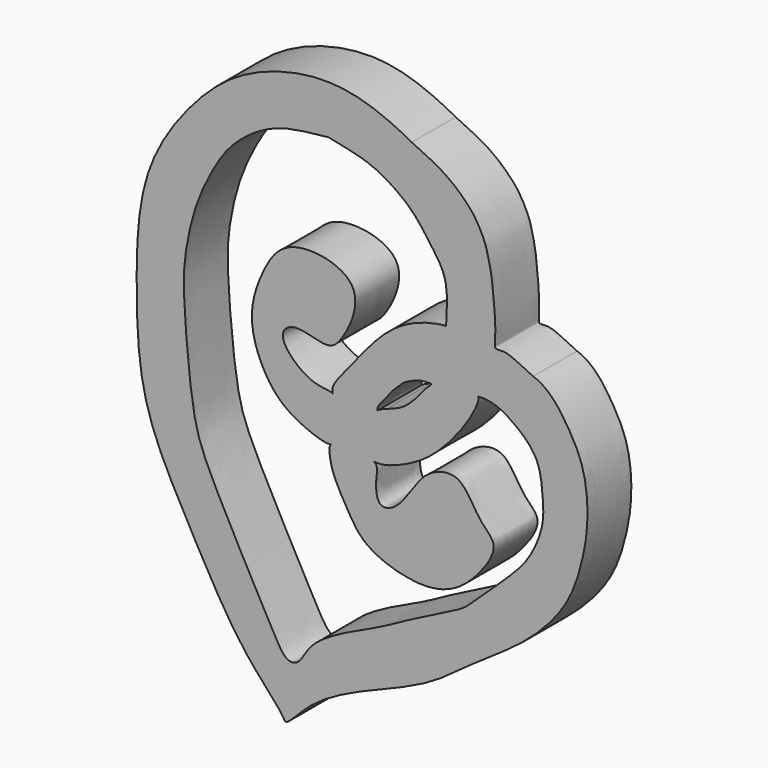
from build123d import *

# Parameters (mm, degrees)
F1_DEPTH = 5.08


with BuildPart() as f1:
    # F0 (on Front) → F1 (new body)
    with BuildSketch(Plane.XZ):
        with BuildLine():
            add(Edge.make_bspline(
                [(12.9434475675, 7.9712104052), (13.7422922583, 7.0552895324), (15.383850226, 7.4895155838), (16.7147424072, 7.0660994388)],
                knots=[0, 0, 0, 0, 0.032523755, 0.032523755, 0.032523755, 0.032523755], degree=3))
            add(Edge.make_bspline(
                [(5.4742157617, 22.5000154136), (7.1555189659, 21.5835338766), (10.6079264327, 19.2692823236), (12.792965037, 16.3012717327), (11.8126951939, 9.2676823139), (12.9434475675, 7.9712104052)],
                knots=[0.8891292206, 0.8891292206, 0.8891292206, 0.8891292206, 0.9190816899, 0.953963125, 1, 1, 1, 1], degree=3))
            add(Edge.make_bspline(
                [(16.7147424072, 7.0660994388), (18.1705162912, 6.6029528559), (20.2002028353, 3.814582201), (21.6276154231, 0.7024454413), (21.878625851, -3.3195361715), (21.2433984405, -6.8677651224), (19.8929255019, -10.9606617131), (15.8219732338, -15.1508443216), (11.9059849161, -17.5286027662), (8.1819090495, -20.4691639784), (4.3745709963, -22.4656705166), (-3.4673550639, -25.2777475035), (-6.167744379, -29.0100693047), (-6.5106842161, -27.9114880188), (-9.5347384807, -24.8231598988), (-12.2070153118, -20.8819726602), (-15.6610498633, -14.5370892856), (-19.7546022552, -6.9166280429), (-20.1138235132, 2.2984539167), (-19.8705389779, 11.9562072399), (-15.278074064, 18.890101701), (-10.4891420475, 23.2536387617), (-3.9979098859, 25.2663354367), (0.8739724373, 24.7488313876), (4.4021569327, 23.0843966965), (5.4742157617, 22.5000154136)],
                knots=[0.032523755, 0.032523755, 0.032523755, 0.032523755, 0.0680993139, 0.0991312099, 0.1315716129, 0.1628613037, 0.196827809, 0.236289651, 0.2721081581, 0.3071300006, 0.3419332968, 0.3906383827, 0.4218035991, 0.4338969606, 0.4674419223, 0.5045569221, 0.5486701725, 0.5970470533, 0.6471152509, 0.6981266005, 0.7448253301, 0.78652913, 0.8282672434, 0.8700304589, 0.8891292206, 0.8891292206, 0.8891292206, 0.8891292206], degree=3))
        make_face()
        with BuildLine():
            add(Edge.make_bspline(
                [(9.0967267751, 8.4237661214), (9.7069410751, 10.3688971985), (9.3624503168, 13.3425321942), (7.5865512086, 15.6957624178), (2.4737122894, 21.0601027649), (-0.723359108, 20.5705333992), (-2.2438063755, 20.398713648)],
                knots=[0, 0, 0, 0, 0.0368945944, 0.0659817142, 0.1101300123, 0.1459332556, 0.1459332556, 0.1459332556, 0.1459332556], degree=3))
            add(Edge.make_bspline(
                [(9.0967267751, 8.4237661214), (9.1872830239, 8.3111572264), (9.0681882989, 8.1135522795), (8.8912698228, 7.8312355092)],
                knots=[0.4443179154, 0.4443179154, 0.4443179154, 0.4443179154, 0.4846199148, 0.4846199148, 0.4846199148, 0.4846199148], degree=3))
            add(Edge.make_bspline(
                [(8.1878295542, 6.1687122103), (8.4276217366, 6.7047841314), (8.6811453239, 7.2721646139), (8.8912698228, 7.8312355092)],
                knots=[0.9858997333, 0.9858997333, 0.9858997333, 0.9858997333, 0.9962963428, 0.9962963428, 0.9962963428, 0.9962963428], degree=3))
            add(Edge.make_bspline(
                [(8.1878295542, 6.1687122103), (7.9519461393, 5.0983688069), (7.8984629879, 3.8675557621), (7.4740075511, 3.4131261086)],
                knots=[0.5409332024, 0.5409332024, 0.5409332024, 0.5409332024, 0.62901496, 0.62901496, 0.62901496, 0.62901496], degree=3))
            add(Edge.make_bspline(
                [(11.6040781144, 3.7775444798), (11.477478549, 3.9287928754), (10.5416642667, 3.5638397897), (8.9438364915, 3.5797258967), (7.9210026078, 3.6470259541), (7.4740075511, 3.4131261086)],
                knots=[0.4067747328, 0.4067747328, 0.4067747328, 0.4067747328, 0.4604712364, 0.5331639229, 0.600084085, 0.600084085, 0.600084085, 0.600084085], degree=3))
            add(Edge.make_bspline(
                [(-2.2438063755, 20.398713648), (-3.7819989375, 20.224888571), (-6.8220176706, 19.9910669526), (-9.8797703177, 18.1168573882), (-11.812113507, 16.2765180291), (-13.4444724283, 13.4822315791), (-14.8338814066, 10.2865686751), (-15.6813672061, 5.915829452), (-15.6718048809, 2.7059369547), (-14.9290377763, -6.2693506201), (-13.4820392885, -10.3627665386), (-7.7791336314, -20.7900216933), (-6.2275032167, -23.7043743852), (-4.7382841994, -23.3833187142), (-4.0116352012, -20.7777478604), (2.824962194, -17.9580007864), (3.716896785, -17.2306321515), (10.0375567411, -14.1751357177), (10.7691950561, -13.4926255954), (14.8620469506, -9.6812376421), (16.4400359685, -7.862924936), (17.7782814094, -4.8688079952), (17.5987993114, -2.3847821386), (17.3248237757, 0.6568030056), (14.8152209906, 2.8605684796), (12.9976128942, 3.8612308109), (11.6040781144, 3.7775444798)],
                knots=[0.1459332556, 0.1459332556, 0.1459332556, 0.1459332556, 0.1821543621, 0.2135270595, 0.2408184896, 0.2706810267, 0.3026577533, 0.337263182, 0.3686746682, 0.4176643155, 0.4558720272, 0.5138481612, 0.5426595154, 0.5588178858, 0.5854633115, 0.6296839427, 0.6521109106, 0.694843456, 0.7150408388, 0.7534868015, 0.7813799803, 0.8106293525, 0.8374214288, 0.8660693306, 0.8958413494, 0.9269237582, 0.9269237582, 0.9269237582, 0.9269237582], degree=3))
        make_face(mode=Mode.SUBTRACT)
        with BuildLine():
            add(Edge.make_bspline(
                [(1.744488909, -4.5375019388), (0.8677657326, -4.1725261398), (-1.1165877802, -4.1685723882), (-1.8031777586, -4.4715595432)],
                knots=[0.9337541015, 0.9337541015, 0.9337541015, 0.9337541015, 1, 1, 1, 1], degree=3))
            add(Edge.make_bspline(
                [(-1.8031777586, -4.4715595432), (-1.8404559451, -4.5218687655), (-1.9006442707, -4.5566302305), (-1.979878497, -4.5776517812)],
                knots=[0, 0, 0, 0, 0.0093101506, 0.0093101506, 0.0093101506, 0.0093101506], degree=3))
            add(Edge.make_bspline(
                [(-1.979878497, -4.5776517812), (-2.146021277, -4.716740037), (-2.1925637655, -5.25566125), (-1.9078192507, -6.9528509723), (-0.403720935, -9.5200361407), (1.1024497908, -12.0904717018), (5.9698548069, -13.5909916524), (9.276599084, -12.9491526932), (11.6185507007, -10.9315279312), (13.76010128, -7.7589194164), (11.552169362, -6.3913693678), (10.0931389819, -2.8303683478), (6.9302755238, -3.7958015432), (5.6477683482, -5.5648613441), (4.0514665571, -7.9919223412), (2.1694807148, -8.2930380541), (2.1078713866, -5.871753229), (2.3717293581, -4.9180660729), (1.9512213842, -4.6439997454)],
                knots=[0.0069872817, 0.0069872817, 0.0069872817, 0.0069872817, 0.0320592076, 0.0809280957, 0.1450863675, 0.2088794877, 0.2903856989, 0.3574745355, 0.4236702519, 0.4896201918, 0.5437921697, 0.6123420385, 0.6714892327, 0.7279590727, 0.7909316087, 0.8325653872, 0.8856045843, 0.927836012, 0.927836012, 0.927836012, 0.927836012], degree=3))
            add(Edge.make_bspline(
                [(1.744488909, -4.5375019388), (1.803345129, -4.5832576861), (1.8727532468, -4.6184021256), (1.9512213842, -4.6439997454)],
                knots=[0.0044131286, 0.0044131286, 0.0044131286, 0.0044131286, 0.0145414142, 0.0145414142, 0.0145414142, 0.0145414142], degree=3))
        make_face()
        with BuildLine():
            add(Edge.make_bspline(
                [(-1.7579157138, -0.4739991861), (-1.6405143241, -0.7798892701), (-2.882157981, -2.3349896326), (-1.5683680299, -4.1546692657), (-1.8031777586, -4.4715595432)],
                knots=[0.8857175032, 0.8857175032, 0.8857175032, 0.8857175032, 0.9413567518, 1, 1, 1, 1], degree=3))
            add(Edge.make_bspline(
                [(-1.7579157138, -0.4739991861), (-1.7857845561, -0.4457267794), (-1.8089843102, -0.4155614822), (-1.8278075546, -0.3836305383)],
                knots=[0, 0, 0, 0, 0.0055635331, 0.0055635331, 0.0055635331, 0.0055635331], degree=3))
            add(Edge.make_bspline(
                [(-1.979878497, -4.5776517812), (-2.5201631579, -4.7209941468), (-5.709785766, -3.6125301156), (-8.0919908162, -1.3152249443), (-9.892318063, 3.2756686057), (-8.4291106971, 7.6044533422), (-6.0293395893, 11.3725496958), (1.8272435626, 9.874669536), (-0.930824539, 4.1182200569), (-2.4017982853, 3.0468672357), (-5.3662148015, 4.3622845997), (-7.3002610522, 2.7073335898), (-4.008367442, -0.3972096502), (-2.0696477036, -0.198188239), (-1.8278075546, -0.3836305383)],
                knots=[0.0093101506, 0.0093101506, 0.0093101506, 0.0093101506, 0.0727944781, 0.1513243107, 0.2363254873, 0.3203813039, 0.4007704635, 0.4952133406, 0.5817297964, 0.6336369718, 0.701644784, 0.7508728854, 0.8307288933, 0.879202819, 0.879202819, 0.879202819, 0.879202819], degree=3))
            add(Edge.make_bspline(
                [(-1.8031777586, -4.4715595432), (-1.8755957909, -4.5035170932), (-1.9335762537, -4.5388893489), (-1.979878497, -4.5776517812)],
                knots=[0, 0, 0, 0, 0.0069872817, 0.0069872817, 0.0069872817, 0.0069872817], degree=3))
        make_face()
        with BuildLine():
            add(Edge.make_bspline(
                [(-1.8278075546, -0.3836305383), (-1.7953052931, -0.4085531748), (-1.7716619991, -0.4381831504), (-1.7579157138, -0.4739991861)],
                knots=[0.879202819, 0.879202819, 0.879202819, 0.879202819, 0.8857175032, 0.8857175032, 0.8857175032, 0.8857175032], degree=3))
            add(Edge.make_bspline(
                [(2.3102690265, -0.3935788376), (0.9132157908, -0.8697028836), (-1.2372399352, -1.0022147899), (-1.7579157138, -0.4739991861)],
                knots=[0.8960560721, 0.8960560721, 0.8960560721, 0.8960560721, 1, 1, 1, 1], degree=3))
            add(Edge.make_bspline(
                [(2.3102690265, -0.3935788376), (2.3015133476, -0.3264421477), (2.2807161141, -0.16697337), (2.4959470425, 0.2023034541), (2.8332862832, 0.627521192), (3.3035486755, 1.1874585024), (3.6341437843, 1.6253036501), (4.327502156, 2.3005659752), (4.5921245208, 2.5574437721), (4.8613102163, 2.746603002), (5.3628034531, 3.0158902117), (5.7337093938, 3.155444778), (6.4055800983, 3.3718904366), (6.7791361032, 3.38399349), (7.3895491313, 3.4302530419), (7.2446144262, 3.2828315968), (7.1890192765, 3.2262825646)],
                knots=[0, 0, 0, 0, 0.048112624, 0.1142811977, 0.1930666071, 0.2810757592, 0.3614890412, 0.4633581969, 0.5267659163, 0.5857978813, 0.6634177515, 0.731855846, 0.8170668919, 0.8877180691, 0.9569300482, 1, 1, 1, 1], degree=3))
            add(Edge.make_bspline(
                [(7.4740075511, 3.4131261086), (7.3771313095, 3.3624335168), (7.2822878055, 3.2992392111), (7.1890192765, 3.2262825646)],
                knots=[0.600084085, 0.600084085, 0.600084085, 0.600084085, 0.6145875424, 0.6145875424, 0.6145875424, 0.6145875424], degree=3))
            add(Edge.make_bspline(
                [(7.4740075511, 3.4131261086), (7.1291072241, 3.8052925292), (7.6199644355, 4.8992106691), (8.1878295542, 6.1687122103)],
                knots=[0.9612789478, 0.9612789478, 0.9612789478, 0.9612789478, 0.9858997333, 0.9858997333, 0.9858997333, 0.9858997333], degree=3))
            add(Edge.make_bspline(
                [(8.8912698228, 7.8312355092), (8.7443724115, 7.5968247023), (8.4300813424, 7.1040674235), (8.2490221942, 6.4463796274), (8.1878295542, 6.1687122103)],
                knots=[0.4846199148, 0.4846199148, 0.4846199148, 0.4846199148, 0.5180831207, 0.5409332024, 0.5409332024, 0.5409332024, 0.5409332024], degree=3))
            add(Edge.make_bspline(
                [(8.8912698228, 7.8312355092), (8.9661239491, 8.0303972616), (9.035470522, 8.2285044873), (9.0967267751, 8.4237661214)],
                knots=[0.9962963428, 0.9962963428, 0.9962963428, 0.9962963428, 1, 1, 1, 1], degree=3))
            add(Edge.make_bspline(
                [(8.6528882261, 8.5413210223), (8.8770312131, 8.5375170606), (9.0352269363, 8.5002426648), (9.0967267751, 8.4237661214)],
                knots=[0.4169474523, 0.4169474523, 0.4169474523, 0.4169474523, 0.4443179154, 0.4443179154, 0.4443179154, 0.4443179154], degree=3))
            add(Edge.make_bspline(
                [(-1.8278075546, -0.3836305383), (-2.1407129568, 0.1471687553), (-0.1034026768, 2.4622539742), (2.0274359286, 5.3457828035), (4.9928557529, 7.8816766991), (8.0166628772, 8.5521184907), (8.6528882261, 8.5413210223)],
                knots=[0.0055635331, 0.0055635331, 0.0055635331, 0.0055635331, 0.0980480978, 0.215740624, 0.3392569447, 0.4169474523, 0.4169474523, 0.4169474523, 0.4169474523], degree=3))
        make_face()
        with BuildLine():
            add(Edge.make_bspline(
                [(3.1468981293, 0), (2.931951581, -0.1477729586), (2.6424011492, -0.2803862363), (2.3102690265, -0.3935788376)],
                knots=[0.8713446892, 0.8713446892, 0.8713446892, 0.8713446892, 0.8960560721, 0.8960560721, 0.8960560721, 0.8960560721], degree=3))
            add(Edge.make_bspline(
                [(2.3102690265, -0.3935788376), (2.2891118291, -0.4098954773), (1.971742302, -0.6758503244), (2.0399786517, -1.5629956952), (1.21914474, -3.9633726364), (1.6736872489, -4.4715595432)],
                knots=[0.8411924098, 0.8411924098, 0.8411924098, 0.8411924098, 0.8453026302, 0.9067646188, 1, 1, 1, 1], degree=3))
            add(Edge.make_bspline(
                [(1.6736872489, -4.4715595432), (1.6952021989, -4.495613654), (1.7188438904, -4.5175650996), (1.744488909, -4.5375019388)],
                knots=[0, 0, 0, 0, 0.0044131286, 0.0044131286, 0.0044131286, 0.0044131286], degree=3))
            add(Edge.make_bspline(
                [(1.9512213842, -4.6439997454), (1.8922936141, -4.6055935355), (1.8228111359, -4.5701071192), (1.744488909, -4.5375019388)],
                knots=[0.927836012, 0.927836012, 0.927836012, 0.927836012, 0.9337541015, 0.9337541015, 0.9337541015, 0.9337541015], degree=3))
            add(Edge.make_bspline(
                [(1.9512213842, -4.6439997454), (2.6340703917, -4.866756521), (5.6580125852, -3.7618111603), (8.1559819998, -1.8426201103), (10.7190482079, 1.2374621807), (11.8005710941, 3.5427944801), (11.6040781144, 3.7775444798)],
                knots=[0.0145414142, 0.0145414142, 0.0145414142, 0.0145414142, 0.1026802428, 0.2092348396, 0.323433325, 0.4067747328, 0.4067747328, 0.4067747328, 0.4067747328], degree=3))
            add(Edge.make_bspline(
                [(11.6040781144, 3.7775444798), (10.0638129481, 3.6850465082), (7.955272299, 2.8659075101), (7.4740075511, 3.4131261086)],
                knots=[0.9269237582, 0.9269237582, 0.9269237582, 0.9269237582, 0.9612789478, 0.9612789478, 0.9612789478, 0.9612789478], degree=3))
            add(Edge.make_bspline(
                [(7.4740075511, 3.4131261086), (7.3918812609, 3.3252002196), (7.2958669077, 3.2663397401), (7.1890192765, 3.2262825646)],
                knots=[0.62901496, 0.62901496, 0.62901496, 0.62901496, 0.6460575689, 0.6460575689, 0.6460575689, 0.6460575689], degree=3))
            add(Edge.make_bspline(
                [(7.1890192765, 3.2262825646), (6.7593736336, 2.8902045151), (5.868035884, 1.6681491471), (4.6775838255, 0.5195748672), (3.4870370119, 0.1231265872), (3.1468981293, 0)],
                knots=[0.6145875424, 0.6145875424, 0.6145875424, 0.6145875424, 0.6813983666, 0.7648837608, 0.8031922007, 0.8031922007, 0.8031922007, 0.8031922007], degree=3))
        make_face()
        with BuildLine():
            add(Edge.make_bspline(
                [(2.3102690265, -0.3935788376), (0.9132157908, -0.8697028836), (-1.2372399352, -1.0022147899), (-1.7579157138, -0.4739991861)],
                knots=[0.8960560721, 0.8960560721, 0.8960560721, 0.8960560721, 1, 1, 1, 1], degree=3))
            add(Edge.make_bspline(
                [(-1.7579157138, -0.4739991861), (-1.6405143241, -0.7798892701), (-2.882157981, -2.3349896326), (-1.5683680299, -4.1546692657), (-1.8031777586, -4.4715595432)],
                knots=[0.8857175032, 0.8857175032, 0.8857175032, 0.8857175032, 0.9413567518, 1, 1, 1, 1], degree=3))
            add(Edge.make_bspline(
                [(1.744488909, -4.5375019388), (0.8677657326, -4.1725261398), (-1.1165877802, -4.1685723882), (-1.8031777586, -4.4715595432)],
                knots=[0.9337541015, 0.9337541015, 0.9337541015, 0.9337541015, 1, 1, 1, 1], degree=3))
            add(Edge.make_bspline(
                [(1.6736872489, -4.4715595432), (1.6952021989, -4.495613654), (1.7188438904, -4.5175650996), (1.744488909, -4.5375019388)],
                knots=[0, 0, 0, 0, 0.0044131286, 0.0044131286, 0.0044131286, 0.0044131286], degree=3))
            add(Edge.make_bspline(
                [(2.3102690265, -0.3935788376), (2.2891118291, -0.4098954773), (1.971742302, -0.6758503244), (2.0399786517, -1.5629956952), (1.21914474, -3.9633726364), (1.6736872489, -4.4715595432)],
                knots=[0.8411924098, 0.8411924098, 0.8411924098, 0.8411924098, 0.8453026302, 0.9067646188, 1, 1, 1, 1], degree=3))
        make_face()
        with BuildLine():
            add(Edge.make_bspline(
                [(8.6528882261, 8.5413210223), (8.6573118025, 8.764038379), (8.6700982482, 9.4105376627), (8.9010512795, 12.5120811805), (7.1446185412, 14.7677796511), (5.5182396397, 17.1994777703), (2.3261182047, 19.2999381018), (0.0475557452, 19.9338278093), (-1.4849121292, 20.2447450015), (-2.2438063755, 20.398713648)],
                knots=[0, 0, 0, 0, 0.0821923834, 0.2379151781, 0.3906147434, 0.5468398096, 0.7220881909, 0.8623514019, 1, 1, 1, 1], degree=3))
            add(Edge.make_bspline(
                [(8.6528882261, 8.5413210223), (8.8770312131, 8.5375170606), (9.0352269363, 8.5002426648), (9.0967267751, 8.4237661214)],
                knots=[0.4169474523, 0.4169474523, 0.4169474523, 0.4169474523, 0.4443179154, 0.4443179154, 0.4443179154, 0.4443179154], degree=3))
            add(Edge.make_bspline(
                [(9.0967267751, 8.4237661214), (9.7069410751, 10.3688971985), (9.3624503168, 13.3425321942), (7.5865512086, 15.6957624178), (2.4737122894, 21.0601027649), (-0.723359108, 20.5705333992), (-2.2438063755, 20.398713648)],
                knots=[0, 0, 0, 0, 0.0368945944, 0.0659817142, 0.1101300123, 0.1459332556, 0.1459332556, 0.1459332556, 0.1459332556], degree=3))
        make_face()
        with BuildLine():
            add(Edge.make_bspline(
                [(5.4742157617, 22.5000154136), (7.1555189659, 21.5835338766), (10.6079264327, 19.2692823236), (12.792965037, 16.3012717327), (11.8126951939, 9.2676823139), (12.9434475675, 7.9712104052)],
                knots=[0.8891292206, 0.8891292206, 0.8891292206, 0.8891292206, 0.9190816899, 0.953963125, 1, 1, 1, 1], degree=3))
            add(Edge.make_bspline(
                [(12.9434475675, 7.9712104052), (13.7422922583, 7.0552895324), (15.383850226, 7.4895155838), (16.7147424072, 7.0660994388)],
                knots=[0, 0, 0, 0, 0.032523755, 0.032523755, 0.032523755, 0.032523755], degree=3))
            add(Edge.make_bspline(
                [(5.4742157617, 22.5000154136), (6.6048410807, 21.9818635579), (8.6490692728, 21.025327604), (10.4856235733, 19.3304707963), (11.356435302, 18.3176420356), (12.2265285656, 16.7109611742), (12.5094360307, 15.650730737), (12.9402160784, 13.9780720862), (13.2292736889, 10.3120608325), (13.2114050623, 9.6254933886), (13.1461194399, 8.4118788475), (13.2400934952, 8.1244857275), (13.9681184874, 8.2567923399), (14.8502028926, 7.989792145), (16.0144664232, 7.4130160971), (16.7147424072, 7.0660994388)],
                knots=[0, 0, 0, 0, 0.1195713442, 0.2170853235, 0.2906566812, 0.3742218826, 0.4391532056, 0.5242501548, 0.6437905361, 0.7011929757, 0.768204249, 0.7977241252, 0.8470768871, 0.9080211414, 1, 1, 1, 1], degree=3))
        make_face()
        with BuildLine():
            add(Edge.make_bspline(
                [(7.4740075511, 3.4131261086), (7.1291072241, 3.8052925292), (7.6199644355, 4.8992106691), (8.1878295542, 6.1687122103)],
                knots=[0.9612789478, 0.9612789478, 0.9612789478, 0.9612789478, 0.9858997333, 0.9858997333, 0.9858997333, 0.9858997333], degree=3))
            add(Edge.make_bspline(
                [(8.1878295542, 6.1687122103), (7.9519461393, 5.0983688069), (7.8984629879, 3.8675557621), (7.4740075511, 3.4131261086)],
                knots=[0.5409332024, 0.5409332024, 0.5409332024, 0.5409332024, 0.62901496, 0.62901496, 0.62901496, 0.62901496], degree=3))
        make_face()
        with BuildLine():
            add(Edge.make_bspline(
                [(11.6040781144, 3.7775444798), (11.477478549, 3.9287928754), (10.5416642667, 3.5638397897), (8.9438364915, 3.5797258967), (7.9210026078, 3.6470259541), (7.4740075511, 3.4131261086)],
                knots=[0.4067747328, 0.4067747328, 0.4067747328, 0.4067747328, 0.4604712364, 0.5331639229, 0.600084085, 0.600084085, 0.600084085, 0.600084085], degree=3))
            add(Edge.make_bspline(
                [(11.6040781144, 3.7775444798), (10.0638129481, 3.6850465082), (7.955272299, 2.8659075101), (7.4740075511, 3.4131261086)],
                knots=[0.9269237582, 0.9269237582, 0.9269237582, 0.9269237582, 0.9612789478, 0.9612789478, 0.9612789478, 0.9612789478], degree=3))
        make_face()
        with BuildLine():
            add(Edge.make_bspline(
                [(8.1878295542, 6.1687122103), (8.4276217366, 6.7047841314), (8.6811453239, 7.2721646139), (8.8912698228, 7.8312355092)],
                knots=[0.9858997333, 0.9858997333, 0.9858997333, 0.9858997333, 0.9962963428, 0.9962963428, 0.9962963428, 0.9962963428], degree=3))
            add(Edge.make_bspline(
                [(8.8912698228, 7.8312355092), (8.7443724115, 7.5968247023), (8.4300813424, 7.1040674235), (8.2490221942, 6.4463796274), (8.1878295542, 6.1687122103)],
                knots=[0.4846199148, 0.4846199148, 0.4846199148, 0.4846199148, 0.5180831207, 0.5409332024, 0.5409332024, 0.5409332024, 0.5409332024], degree=3))
        make_face()
        with BuildLine():
            add(Edge.make_bspline(
                [(3.1468981293, 0), (2.8094960148, -0.1221359069), (2.5058736029, -0.2427266561), (2.3102690265, -0.3935788376)],
                knots=[0.8031922007, 0.8031922007, 0.8031922007, 0.8031922007, 0.8411924098, 0.8411924098, 0.8411924098, 0.8411924098], degree=3))
            add(Edge.make_bspline(
                [(3.1468981293, 0), (2.931951581, -0.1477729586), (2.6424011492, -0.2803862363), (2.3102690265, -0.3935788376)],
                knots=[0.8713446892, 0.8713446892, 0.8713446892, 0.8713446892, 0.8960560721, 0.8960560721, 0.8960560721, 0.8960560721], degree=3))
        make_face()
        with BuildLine():
            add(Edge.make_bspline(
                [(9.0967267751, 8.4237661214), (9.1872830239, 8.3111572264), (9.0681882989, 8.1135522795), (8.8912698228, 7.8312355092)],
                knots=[0.4443179154, 0.4443179154, 0.4443179154, 0.4443179154, 0.4846199148, 0.4846199148, 0.4846199148, 0.4846199148], degree=3))
            add(Edge.make_bspline(
                [(8.8912698228, 7.8312355092), (8.9661239491, 8.0303972616), (9.035470522, 8.2285044873), (9.0967267751, 8.4237661214)],
                knots=[0.9962963428, 0.9962963428, 0.9962963428, 0.9962963428, 1, 1, 1, 1], degree=3))
        make_face()
        with BuildLine():
            add(Edge.make_bspline(
                [(7.4740075511, 3.4131261086), (7.3771313095, 3.3624335168), (7.2822878055, 3.2992392111), (7.1890192765, 3.2262825646)],
                knots=[0.600084085, 0.600084085, 0.600084085, 0.600084085, 0.6145875424, 0.6145875424, 0.6145875424, 0.6145875424], degree=3))
            add(Edge.make_bspline(
                [(7.4740075511, 3.4131261086), (7.3918812609, 3.3252002196), (7.2958669077, 3.2663397401), (7.1890192765, 3.2262825646)],
                knots=[0.62901496, 0.62901496, 0.62901496, 0.62901496, 0.6460575689, 0.6460575689, 0.6460575689, 0.6460575689], degree=3))
        make_face()
        with BuildLine():
            add(Edge.make_bspline(
                [(-1.8031777586, -4.4715595432), (-1.8404559451, -4.5218687655), (-1.9006442707, -4.5566302305), (-1.979878497, -4.5776517812)],
                knots=[0, 0, 0, 0, 0.0093101506, 0.0093101506, 0.0093101506, 0.0093101506], degree=3))
            add(Edge.make_bspline(
                [(-1.8031777586, -4.4715595432), (-1.8755957909, -4.5035170932), (-1.9335762537, -4.5388893489), (-1.979878497, -4.5776517812)],
                knots=[0, 0, 0, 0, 0.0069872817, 0.0069872817, 0.0069872817, 0.0069872817], degree=3))
        make_face()
        with BuildLine():
            add(Edge.make_bspline(
                [(1.9512213842, -4.6439997454), (1.8922936141, -4.6055935355), (1.8228111359, -4.5701071192), (1.744488909, -4.5375019388)],
                knots=[0.927836012, 0.927836012, 0.927836012, 0.927836012, 0.9337541015, 0.9337541015, 0.9337541015, 0.9337541015], degree=3))
            add(Edge.make_bspline(
                [(1.744488909, -4.5375019388), (1.803345129, -4.5832576861), (1.8727532468, -4.6184021256), (1.9512213842, -4.6439997454)],
                knots=[0.0044131286, 0.0044131286, 0.0044131286, 0.0044131286, 0.0145414142, 0.0145414142, 0.0145414142, 0.0145414142], degree=3))
        make_face()
        with BuildLine():
            add(Edge.make_bspline(
                [(-1.7579157138, -0.4739991861), (-1.7857845561, -0.4457267794), (-1.8089843102, -0.4155614822), (-1.8278075546, -0.3836305383)],
                knots=[0, 0, 0, 0, 0.0055635331, 0.0055635331, 0.0055635331, 0.0055635331], degree=3))
            add(Edge.make_bspline(
                [(-1.8278075546, -0.3836305383), (-1.7953052931, -0.4085531748), (-1.7716619991, -0.4381831504), (-1.7579157138, -0.4739991861)],
                knots=[0.879202819, 0.879202819, 0.879202819, 0.879202819, 0.8857175032, 0.8857175032, 0.8857175032, 0.8857175032], degree=3))
        make_face()
    extrude(amount=F1_DEPTH)


solid = f1.part
